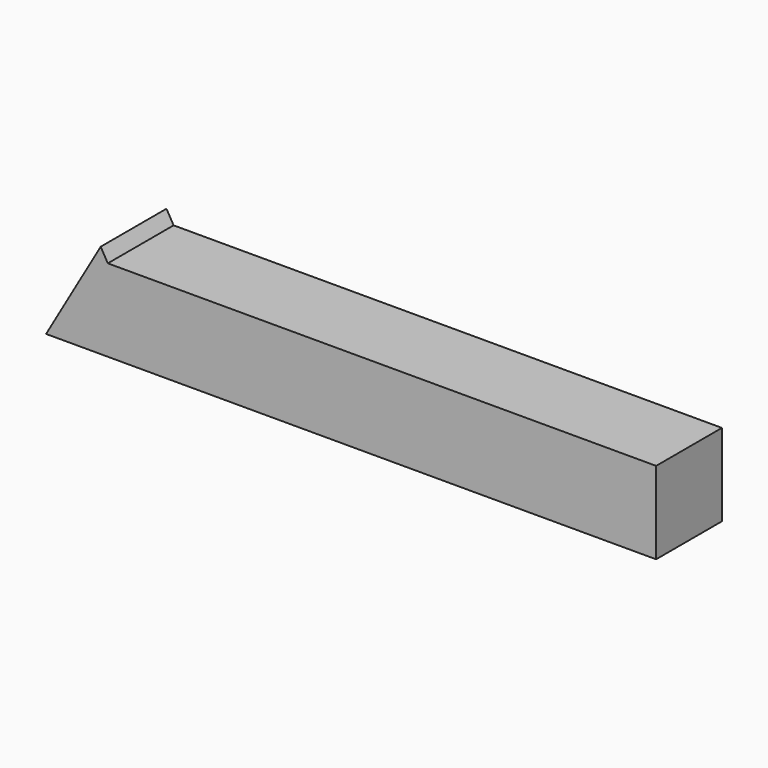
from build123d import *

# Parameters (mm, degrees)
F1_DEPTH = 12


# Not quite as in the source:
# - a feature names something its author has since deleted; it is built from what else it names


with BuildPart() as f1:
    # F0 (on Front) → F1 (new body)
    with BuildSketch(Plane.XZ):
        Polygon((7.9674337148, 13.8), (0, 0), (89, 0), (89, 12), (9.0066641994, 12), align=None)
    extrude(amount=-F1_DEPTH)


solid = f1.part
